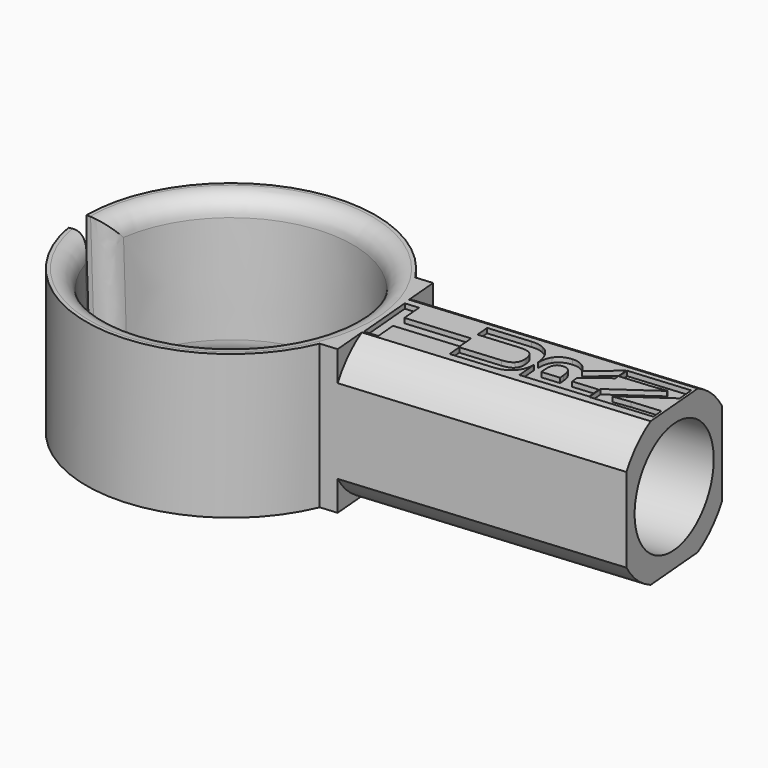
from build123d import *

# Parameters (mm, degrees)
F1_ANGLE        = 350
F3_DEPTH        = 49.276
F4_W            = 35.56
F4_H            = 38.1
F5_DEPTH        = 76.2
F6_R            = 14.732
F7_DEPTH        = 50.8
F8_R            = 26.0582213514
F8_R_2          = 20.9782213514
F9_DEPTH        = 71.628
F10_R           = 5.08
F11_TEXT_SIZE   = 23.8804699611
F11_TEXT_SIZE_2 = 27.123283417
F12_DEPTH       = 1.27
F13_TEXT_SIZE   = 22.2988564439
F13_TEXT_SIZE_2 = 28.1625677553
F14_DEPTH       = 1.27


# Not quite as in the source:
# - Text() gives the source's letters only with a copy of the font that has no kerning and outlines rounded to 1/6400 em; it was checked with that copy


with BuildPart() as f1:
    # F0 (on Front) → F1 (revolve)
    with BuildSketch(Plane.XZ):
        Polygon((-31.115, -7.6052526687), (-32.385, 30.4947473313), (-38.227, 30.4947473313), (-38.227, -7.6052526687), align=None)
    revolve(axis=Axis((0, 0, 1.9106518195), (0, 0, -1)), revolution_arc=F1_ANGLE)

    # F2 (on face) → F3 (cut)
    with BuildSketch(Plane.XY.offset(30.4947473313)):
        with BuildLine():
            Line((33.8455, 0), (35.306, 0))
            Line((35.306, 0), (38.227, 0))
            ThreePointArc((38.227, 0), (38.6644446885, 3.3827005918), (37.6462459744, 6.6380488877))
            Line((37.6462459744, 6.6380488877), (34.7696225278, 6.1308225607))
            Line((34.7696225278, 6.1308225607), (33.3313108046, 5.8772093972))
            Line((33.3313108046, 5.8772093972), (33.8455, 0))
        make_face()
    extrude(amount=-F3_DEPTH, mode=Mode.SUBTRACT)

    # F4 (on face) → F5 (join)
    with BuildSketch(Plane(origin=(33.5884054023, 2.9386046986, 0), x_dir=(-0.0871557427, 0.9961946981, 0), z_dir=(0.9961946981, 0.0871557427, 0))):
        with Locations((0, 11.4447473313)):
            Rectangle(F4_W, F4_H)
    extrude(amount=F5_DEPTH)

    # F6 (on face) → F7 (cut)
    with BuildSketch(Plane(origin=(109.4984413969, 9.579872296, 0), x_dir=(-0.0871557427, 0.9961946981, 0), z_dir=(0.9961946981, 0.0871557427, 0))):
        with Locations((0, 11.4447473313)):
            Circle(F6_R)
    extrude(amount=-F7_DEPTH, mode=Mode.SUBTRACT)

    # F8 (on face) → F9 (cut)
    with BuildSketch(Plane(origin=(109.4984413969, 9.579872296, 0), x_dir=(-0.0871557427, 0.9961946981, 0), z_dir=(0.9961946981, 0.0871557427, 0))):
        with Locations((0, 11.4447473313)):
            Circle(F8_R)
        with Locations((0, 11.4447473313)):
            Circle(F8_R_2, mode=Mode.SUBTRACT)
    extrude(amount=-F9_DEPTH, mode=Mode.SUBTRACT)

    # F10
    f10_edges = [f1.edges().sort_by_distance(p)[0] for p in [
        (-31.75, 0, 11.444747),
        (-31.267646, -5.51333, 11.444747),
        (32.261765, 2.822539, 30.494747),
        (30.996598, 2.711851, -7.605253),
    ]]
    fillet(f10_edges, radius=F10_R)

    # F11 (on face) → F12 (cut)
    with BuildSketch(Plane(origin=(0, 0, -7.6052526687), x_dir=(1, 0, 0), z_dir=(0, 0, -1))):
        with Locations(Location((66.0966437804, -14.6016668518), (0, 0, 85))):
            Text('U', F11_TEXT_SIZE, font='Open Sans', font_style=FontStyle.BOLD, text_align=(TextAlign.LEFT, TextAlign.BOTTOM))
        with Locations(Location((97.1419191216, -17.3177765002), (0, 0, 85))):
            Text('P', F11_TEXT_SIZE_2, font='Open Sans', font_style=FontStyle.BOLD, text_align=(TextAlign.LEFT, TextAlign.BOTTOM))
    extrude(amount=-F12_DEPTH, mode=Mode.SUBTRACT)

    # F13 (on face) → F14 (cut)
    with BuildSketch(Plane.XY.offset(30.4947473313)):
        with Locations(Location((109.6144093009, 0.771058349), (0, 0, 95))):
            Text('N', F13_TEXT_SIZE, font='Open Sans', font_style=FontStyle.BOLD, text_align=(TextAlign.LEFT, TextAlign.BOTTOM))
        with Locations(Location((59.1085942045, -3.6476279141), (0, 0, 95))):
            Text('T', F13_TEXT_SIZE_2, font='Open Sans', font_style=FontStyle.BOLD, text_align=(TextAlign.LEFT, TextAlign.BOTTOM))
        with BuildLine():
            Line((68.8449467368, 13.2876979649), (57.8571263623, 12.3263882453))
            Line((57.8571263623, 12.3263882453), (58.1712756144, 8.7356458631))
            Line((58.1712756144, 8.7356458631), (68.5457704267, 9.643296549))
            add(Edge.make_bspline(
                [(71.5128632081, 9.1013301641), (70.5195635995, 9.8159810758), (68.5457704267, 9.643296549)],
                knots=[0, 0, 0, 1, 1, 1], degree=2))
            add(Edge.make_bspline(
                [(72.6606357927, 6.6210450583), (72.5061628168, 8.3866792525), (71.5128632081, 9.1013301641)],
                knots=[0, 0, 0, 1, 1, 1], degree=2))
            add(Edge.make_bspline(
                [(71.9712886192, 3.9257219412), (72.8203120688, 4.7959368703), (72.6606357927, 6.6210450583)],
                knots=[0, 0, 0, 1, 1, 1], degree=2))
            add(Edge.make_bspline(
                [(69.1596233706, 2.8837981042), (71.1222651696, 3.0555070122), (71.9712886192, 3.9257219412)],
                knots=[0, 0, 0, 1, 1, 1], degree=2))
            Line((69.1596233706, 2.8837981042), (58.7628258106, 1.9741961807))
            Line((58.7628258106, 1.9741961807), (59.0766498564, -1.6128290769))
            Line((59.0766498564, -1.6128290769), (70.0198647355, -0.6554218324))
            add(Edge.make_bspline(
                [(74.4556927106, 1.5586313631), (72.934090437, -0.4004601206), (70.0198647355, -0.6554218324)],
                knots=[0, 0, 0, 1, 1, 1], degree=2))
            add(Edge.make_bspline(
                [(75.7285163289, 5.3938617344), (75.637079006, 3.0796883899), (74.4556927106, 1.5586313631)],
                knots=[0.2235906085, 0.2235906085, 0.2235906085, 1, 1, 1], degree=2))
            add(Edge.make_bspline(
                [(75.7285163289, 5.3938617344), (75.678238352, 6.121268856), (75.6926161259, 6.7714161135)],
                knots=[0.0489190415, 0.0489190415, 0.0489190415, 0.2608825985, 0.2608825985, 0.2608825985], degree=2))
            add(Edge.make_bspline(
                [(75.6907882647, 6.7925096364), (75.6917115846, 6.7819560427), (75.6926161259, 6.7714161135)],
                knots=[0, 0, 0, 0.0032226811, 0.0032226811, 0.0032226811], degree=2))
            add(Edge.make_bspline(
                [(74.6050820613, 10.4899188384), (75.5008678059, 8.963310414), (75.6907882647, 6.7925096364)],
                knots=[0, 0, 0, 1, 1, 1], degree=2))
            add(Edge.make_bspline(
                [(72.2194126177, 12.7345524021), (73.7092963167, 12.0165272628), (74.6050820613, 10.4899188384)],
                knots=[0, 0, 0, 1, 1, 1], degree=2))
            add(Edge.make_bspline(
                [(68.8449467368, 13.2876979649), (70.7295289188, 13.4525775413), (72.2194126177, 12.7345524021)],
                knots=[0, 0, 0, 1, 1, 1], degree=2))
        make_face()
        with BuildLine():
            add(Edge.make_bspline(
                [(75.6926161259, 6.7714161135), (75.7427514561, 9.0384810675), (76.5790480063, 10.3661290599)],
                knots=[0.2608825985, 0.2608825985, 0.2608825985, 1, 1, 1], degree=2))
            add(Edge.make_bspline(
                [(75.6926161259, 6.7714161135), (75.7544689431, 6.0506925108), (75.7285163289, 5.3938617344)],
                knots=[0.0032226811, 0.0032226811, 0.0032226811, 0.2235906085, 0.2235906085, 0.2235906085], degree=2))
            add(Edge.make_bspline(
                [(75.7551674459, 5.0539901795), (75.7401199766, 5.2259835402), (75.7285163289, 5.3938617344)],
                knots=[0, 0, 0, 0.0489190415, 0.0489190415, 0.0489190415], degree=2))
            Line((75.7551674459, 5.0539901795), (76.1944537559, 0.0329246803))
            Line((76.1944537559, 0.0329246803), (93.4305531293, 1.5408879789))
            Line((93.4305531293, 1.5408879789), (93.1107421343, 5.1963443792))
            Line((93.1107421343, 5.1963443792), (86.4977234865, 4.6177802158))
            Line((86.4977234865, 4.6177802158), (86.3277516987, 6.5605666411))
            Line((86.3277516987, 6.5605666411), (92.58069419, 11.2548201055))
            Line((92.58069419, 11.2548201055), (92.2258987104, 15.3101509933))
            add(Edge.make_bspline(
                [(85.1586255261, 9.582930051), (90.6312915384, 13.9846428977), (92.2258987104, 15.3101509933)],
                knots=[0, 0, 0, 1, 1, 1], degree=2))
            add(Edge.make_bspline(
                [(83.0951727301, 11.7915031553), (84.3528109604, 11.0595496566), (85.1586255261, 9.582930051)],
                knots=[0, 0, 0, 1, 1, 1], degree=2))
            add(Edge.make_bspline(
                [(80.3172569671, 12.3904496044), (81.8375344999, 12.5234566539), (83.0951727301, 11.7915031553)],
                knots=[0, 0, 0, 1, 1, 1], degree=2))
            add(Edge.make_bspline(
                [(76.5790480063, 10.3661290599), (77.7105279964, 12.1623903706), (80.3172569671, 12.3904496044)],
                knots=[0, 0, 0, 1, 1, 1], degree=2))
        make_face()
        with BuildLine():
            Line((83.4220984361, 5.5346959359), (83.5250716357, 4.3577068782))
            Line((83.5250716357, 4.3577068782), (78.8699290166, 3.950434672))
            Line((78.8699290166, 3.950434672), (78.7728965785, 5.0595205148))
            add(Edge.make_bspline(
                [(79.0633774371, 7.713516503), (78.618436779, 6.8250041013), (78.7728965785, 5.0595205148)],
                knots=[0, 0, 0, 1, 1, 1], degree=2))
            add(Edge.make_bspline(
                [(80.7343483635, 8.7092926544), (79.5083180951, 8.6020289047), (79.0633774371, 7.713516503)],
                knots=[0, 0, 0, 1, 1, 1], degree=2))
            add(Edge.make_bspline(
                [(82.6209874048, 8.0437734234), (81.9716958344, 8.8175465309), (80.7343483635, 8.7092926544)],
                knots=[0, 0, 0, 1, 1, 1], degree=2))
            add(Edge.make_bspline(
                [(83.4220984361, 5.5346959359), (83.2702789751, 7.2700003158), (82.6209874048, 8.0437734234)],
                knots=[0, 0, 0, 1, 1, 1], degree=2))
        make_face(mode=Mode.SUBTRACT)
        with BuildLine():
            add(Edge.make_bspline(
                [(75.6926161259, 6.7714161135), (75.7544689431, 6.0506925108), (75.7285163289, 5.3938617344)],
                knots=[0.0032226811, 0.0032226811, 0.0032226811, 0.2235906085, 0.2235906085, 0.2235906085], degree=2))
            add(Edge.make_bspline(
                [(75.7285163289, 5.3938617344), (75.678238352, 6.121268856), (75.6926161259, 6.7714161135)],
                knots=[0.0489190415, 0.0489190415, 0.0489190415, 0.2608825985, 0.2608825985, 0.2608825985], degree=2))
        make_face()
    extrude(amount=-F14_DEPTH, mode=Mode.SUBTRACT)


solid = f1.part
